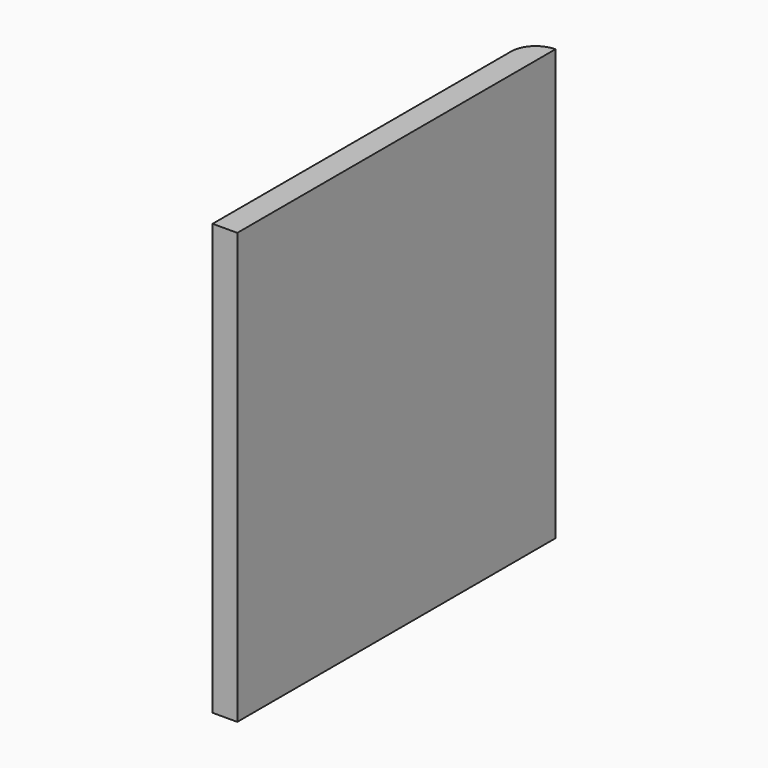
from build123d import *

# Parameters (mm, degrees)
F0_W     = 290
F0_H     = 314
F1_DEPTH = 18
F3_DEPTH = 5
F4_R     = 17.99999


# Not quite as in the source:
# - a fillet or chamfer is up to 0.001 mm smaller than in the source, because OpenCascade refuses the exact size


with BuildPart() as f1:
    # F0 (on Right) → F1 (new body)
    with BuildSketch(Plane.YZ):
        Rectangle(F0_W, F0_H)
    extrude(amount=F1_DEPTH)

    # F2 (on face) → F3 (cut)
    with BuildSketch(Plane(origin=(0, 0, 0), x_dir=(0, -1, 0), z_dir=(-1, 0, 0))):
        with BuildLine():
            Line((28.5, 9), (-28.5, 9))
            ThreePointArc((-28.5, 9), (-37.5, 0), (-28.5, -9))
            Line((-28.5, -9), (28.5, -9))
            ThreePointArc((28.5, -9), (37.5, 0), (28.5, 9))
        make_face()
    extrude(amount=-F3_DEPTH, mode=Mode.SUBTRACT)

    # F4 (radius 18 in the source; OpenCascade refuses exactly that, so slightly less here)
    f4_edges = [f1.edges().sort_by_distance(p)[0] for p in [
        (0, 145, 0),
    ]]
    fillet(f4_edges, radius=F4_R)


solid = f1.part
